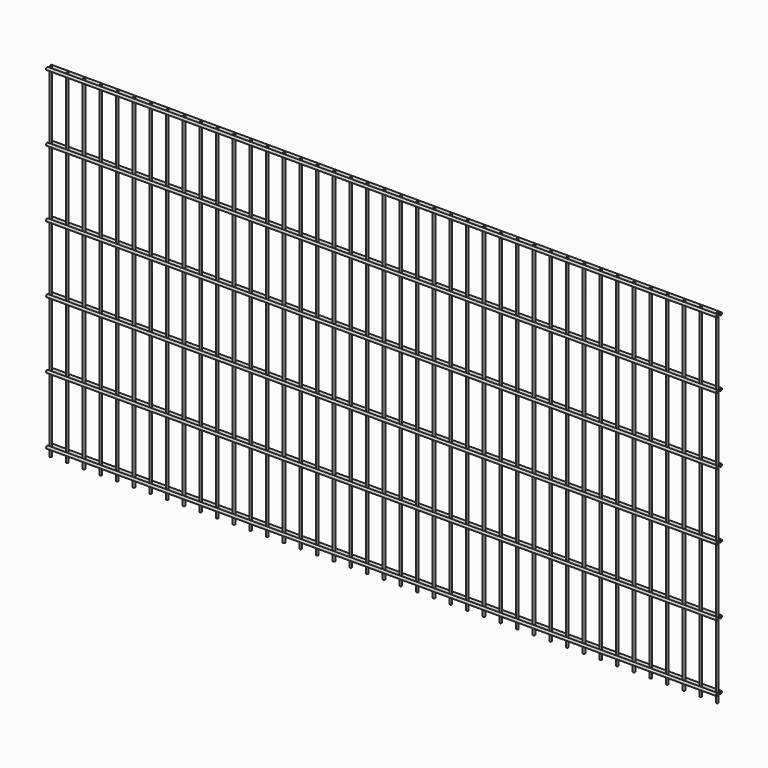
from build123d import *

# Parameters (mm, degrees)
F0_R     = 3
F1_DEPTH = 1030
F2_R     = 4
F3_DEPTH = 1005


with BuildPart() as f1:
    # F0 (on Top) → F1 (new body)
    with BuildSketch(Plane.XY):
        with Locations((750, 0)):
            Circle(F0_R)
    extrude(amount=-F1_DEPTH)


with BuildPart() as f1b:
    # F0 (on Top) → F1, piece 2 (new body)
    with BuildSketch(Plane.XY):
        with Locations((-550, 0)):
            Circle(F0_R)
    extrude(amount=-F1_DEPTH)


with BuildPart() as f1c:
    # F0 (on Top) → F1, piece 3 (new body)
    with BuildSketch(Plane.XY):
        with Locations((950, 0)):
            Circle(F0_R)
    extrude(amount=-F1_DEPTH)


with BuildPart() as f1d:
    # F0 (on Top) → F1, piece 4 (new body)
    with BuildSketch(Plane.XY):
        with Locations((450, 0)):
            Circle(F0_R)
    extrude(amount=-F1_DEPTH)


with BuildPart() as f1e:
    # F0 (on Top) → F1, piece 5 (new body)
    with BuildSketch(Plane.XY):
        with Locations((-800, 0)):
            Circle(F0_R)
    extrude(amount=-F1_DEPTH)


with BuildPart() as f1f:
    # F0 (on Top) → F1, piece 6 (new body)
    with BuildSketch(Plane.XY):
        with Locations((-900, 0)):
            Circle(F0_R)
    extrude(amount=-F1_DEPTH)


with BuildPart() as f1g:
    # F0 (on Top) → F1, piece 7 (new body)
    with BuildSketch(Plane.XY):
        with Locations((350, 0)):
            Circle(F0_R)
    extrude(amount=-F1_DEPTH)


with BuildPart() as f1h:
    # F0 (on Top) → F1, piece 8 (new body)
    with BuildSketch(Plane.XY):
        with Locations((-700, 0)):
            Circle(F0_R)
    extrude(amount=-F1_DEPTH)


with BuildPart() as f1i:
    # F0 (on Top) → F1, piece 9 (new body)
    with BuildSketch(Plane.XY):
        with Locations((1000, 0)):
            Circle(F0_R)
    extrude(amount=-F1_DEPTH)


with BuildPart() as f1j:
    # F0 (on Top) → F1, piece 10 (new body)
    with BuildSketch(Plane.XY):
        with Locations((600, 0)):
            Circle(F0_R)
    extrude(amount=-F1_DEPTH)


with BuildPart() as f1k:
    # F0 (on Top) → F1, piece 11 (new body)
    with BuildSketch(Plane.XY):
        with Locations((700, 0)):
            Circle(F0_R)
    extrude(amount=-F1_DEPTH)


with BuildPart() as f1l:
    # F0 (on Top) → F1, piece 12 (new body)
    with BuildSketch(Plane.XY):
        with Locations((650, 0)):
            Circle(F0_R)
    extrude(amount=-F1_DEPTH)


with BuildPart() as f1m:
    # F0 (on Top) → F1, piece 13 (new body)
    with BuildSketch(Plane.XY):
        with Locations((-650, 0)):
            Circle(F0_R)
    extrude(amount=-F1_DEPTH)


with BuildPart() as f1n:
    # F0 (on Top) → F1, piece 14 (new body)
    with BuildSketch(Plane.XY):
        with Locations((850, 0)):
            Circle(F0_R)
    extrude(amount=-F1_DEPTH)


with BuildPart() as f1o:
    # F0 (on Top) → F1, piece 15 (new body)
    with BuildSketch(Plane.XY):
        with Locations((-300, 0)):
            Circle(F0_R)
    extrude(amount=-F1_DEPTH)


with BuildPart() as f1p:
    # F0 (on Top) → F1, piece 16 (new body)
    with BuildSketch(Plane.XY):
        with Locations((-250, 0)):
            Circle(F0_R)
    extrude(amount=-F1_DEPTH)


with BuildPart() as f1q:
    # F0 (on Top) → F1, piece 17 (new body)
    with BuildSketch(Plane.XY):
        with Locations((-350, 0)):
            Circle(F0_R)
    extrude(amount=-F1_DEPTH)


with BuildPart() as f1r:
    # F0 (on Top) → F1, piece 18 (new body)
    with BuildSketch(Plane.XY):
        with Locations((-400, 0)):
            Circle(F0_R)
    extrude(amount=-F1_DEPTH)


with BuildPart() as f1s:
    # F0 (on Top) → F1, piece 19 (new body)
    with BuildSketch(Plane.XY):
        with Locations((-500, 0)):
            Circle(F0_R)
    extrude(amount=-F1_DEPTH)


with BuildPart() as f1t:
    # F0 (on Top) → F1, piece 20 (new body)
    with BuildSketch(Plane.XY):
        with Locations((-950, 0)):
            Circle(F0_R)
    extrude(amount=-F1_DEPTH)


with BuildPart() as f1u:
    # F0 (on Top) → F1, piece 21 (new body)
    with BuildSketch(Plane.XY):
        with Locations((-450, 0)):
            Circle(F0_R)
    extrude(amount=-F1_DEPTH)


with BuildPart() as f1v:
    # F0 (on Top) → F1, piece 22 (new body)
    with BuildSketch(Plane.XY):
        with Locations((150, 0)):
            Circle(F0_R)
    extrude(amount=-F1_DEPTH)


with BuildPart() as f1w:
    # F0 (on Top) → F1, piece 23 (new body)
    with BuildSketch(Plane.XY):
        with Locations((50, 0)):
            Circle(F0_R)
    extrude(amount=-F1_DEPTH)


with BuildPart() as f1x:
    # F0 (on Top) → F1, piece 24 (new body)
    with BuildSketch(Plane.XY):
        with Locations((100, 0)):
            Circle(F0_R)
    extrude(amount=-F1_DEPTH)


with BuildPart() as f1y:
    # F0 (on Top) → F1, piece 25 (new body)
    with BuildSketch(Plane.XY):
        Circle(F0_R)
    extrude(amount=-F1_DEPTH)


with BuildPart() as f1z:
    # F0 (on Top) → F1, piece 26 (new body)
    with BuildSketch(Plane.XY):
        with Locations((-50, 0)):
            Circle(F0_R)
    extrude(amount=-F1_DEPTH)


with BuildPart() as f1ba:
    # F0 (on Top) → F1, piece 27 (new body)
    with BuildSketch(Plane.XY):
        with Locations((-150, 0)):
            Circle(F0_R)
    extrude(amount=-F1_DEPTH)


with BuildPart() as f1bb:
    # F0 (on Top) → F1, piece 28 (new body)
    with BuildSketch(Plane.XY):
        with Locations((-100, 0)):
            Circle(F0_R)
    extrude(amount=-F1_DEPTH)


with BuildPart() as f1bc:
    # F0 (on Top) → F1, piece 29 (new body)
    with BuildSketch(Plane.XY):
        with Locations((-1000, 0)):
            Circle(F0_R)
    extrude(amount=-F1_DEPTH)


with BuildPart() as f1bd:
    # F0 (on Top) → F1, piece 30 (new body)
    with BuildSketch(Plane.XY):
        with Locations((300, 0)):
            Circle(F0_R)
    extrude(amount=-F1_DEPTH)


with BuildPart() as f1be:
    # F0 (on Top) → F1, piece 31 (new body)
    with BuildSketch(Plane.XY):
        with Locations((250, 0)):
            Circle(F0_R)
    extrude(amount=-F1_DEPTH)


with BuildPart() as f1bf:
    # F0 (on Top) → F1, piece 32 (new body)
    with BuildSketch(Plane.XY):
        with Locations((-200, 0)):
            Circle(F0_R)
    extrude(amount=-F1_DEPTH)


with BuildPart() as f1bg:
    # F0 (on Top) → F1, piece 33 (new body)
    with BuildSketch(Plane.XY):
        with Locations((900, 0)):
            Circle(F0_R)
    extrude(amount=-F1_DEPTH)


with BuildPart() as f1bh:
    # F0 (on Top) → F1, piece 34 (new body)
    with BuildSketch(Plane.XY):
        with Locations((-750, 0)):
            Circle(F0_R)
    extrude(amount=-F1_DEPTH)


with BuildPart() as f1bi:
    # F0 (on Top) → F1, piece 35 (new body)
    with BuildSketch(Plane.XY):
        with Locations((200, 0)):
            Circle(F0_R)
    extrude(amount=-F1_DEPTH)


with BuildPart() as f1bj:
    # F0 (on Top) → F1, piece 36 (new body)
    with BuildSketch(Plane.XY):
        with Locations((500, 0)):
            Circle(F0_R)
    extrude(amount=-F1_DEPTH)


with BuildPart() as f1bk:
    # F0 (on Top) → F1, piece 37 (new body)
    with BuildSketch(Plane.XY):
        with Locations((550, 0)):
            Circle(F0_R)
    extrude(amount=-F1_DEPTH)


with BuildPart() as f1bl:
    # F0 (on Top) → F1, piece 38 (new body)
    with BuildSketch(Plane.XY):
        with Locations((-600, 0)):
            Circle(F0_R)
    extrude(amount=-F1_DEPTH)


with BuildPart() as f1bm:
    # F0 (on Top) → F1, piece 39 (new body)
    with BuildSketch(Plane.XY):
        with Locations((800, 0)):
            Circle(F0_R)
    extrude(amount=-F1_DEPTH)


with BuildPart() as f1bn:
    # F0 (on Top) → F1, piece 40 (new body)
    with BuildSketch(Plane.XY):
        with Locations((-850, 0)):
            Circle(F0_R)
    extrude(amount=-F1_DEPTH)


with BuildPart() as f1bo:
    # F0 (on Top) → F1, piece 41 (new body)
    with BuildSketch(Plane.XY):
        with Locations((400, 0)):
            Circle(F0_R)
    extrude(amount=-F1_DEPTH)


with BuildPart() as f3:
    # F2 (on Right) → F3 (new body, symmetric)
    with BuildSketch(Plane.YZ):
        with Locations((7, -4)):
            Circle(F2_R)
    extrude(amount=F3_DEPTH, both=True)


with BuildPart() as f3b:
    # F2 (on Right) → F3, piece 2 (new body, symmetric)
    with BuildSketch(Plane.YZ):
        with Locations((-7, -4)):
            Circle(F2_R)
    extrude(amount=F3_DEPTH, both=True)


with BuildPart() as f3c:
    # F2 (on Right) → F3, piece 3 (new body, symmetric)
    with BuildSketch(Plane.YZ):
        with Locations((7, -204)):
            Circle(F2_R)
    extrude(amount=F3_DEPTH, both=True)


with BuildPart() as f3d:
    # F2 (on Right) → F3, piece 4 (new body, symmetric)
    with BuildSketch(Plane.YZ):
        with Locations((-7, -204)):
            Circle(F2_R)
    extrude(amount=F3_DEPTH, both=True)


with BuildPart() as f3e:
    # F2 (on Right) → F3, piece 5 (new body, symmetric)
    with BuildSketch(Plane.YZ):
        with Locations((7, -404)):
            Circle(F2_R)
    extrude(amount=F3_DEPTH, both=True)


with BuildPart() as f3f:
    # F2 (on Right) → F3, piece 6 (new body, symmetric)
    with BuildSketch(Plane.YZ):
        with Locations((-7, -404)):
            Circle(F2_R)
    extrude(amount=F3_DEPTH, both=True)


with BuildPart() as f3g:
    # F2 (on Right) → F3, piece 7 (new body, symmetric)
    with BuildSketch(Plane.YZ):
        with Locations((7, -604)):
            Circle(F2_R)
    extrude(amount=F3_DEPTH, both=True)


with BuildPart() as f3h:
    # F2 (on Right) → F3, piece 8 (new body, symmetric)
    with BuildSketch(Plane.YZ):
        with Locations((-7, -604)):
            Circle(F2_R)
    extrude(amount=F3_DEPTH, both=True)


with BuildPart() as f3i:
    # F2 (on Right) → F3, piece 9 (new body, symmetric)
    with BuildSketch(Plane.YZ):
        with Locations((7, -804)):
            Circle(F2_R)
    extrude(amount=F3_DEPTH, both=True)


with BuildPart() as f3j:
    # F2 (on Right) → F3, piece 10 (new body, symmetric)
    with BuildSketch(Plane.YZ):
        with Locations((-7, -804)):
            Circle(F2_R)
    extrude(amount=F3_DEPTH, both=True)


with BuildPart() as f3k:
    # F2 (on Right) → F3, piece 11 (new body, symmetric)
    with BuildSketch(Plane.YZ):
        with Locations((7, -1004)):
            Circle(F2_R)
    extrude(amount=F3_DEPTH, both=True)


with BuildPart() as f3l:
    # F2 (on Right) → F3, piece 12 (new body, symmetric)
    with BuildSketch(Plane.YZ):
        with Locations((-7, -1004)):
            Circle(F2_R)
    extrude(amount=F3_DEPTH, both=True)


solid = Compound([f1.part, f1b.part, f1c.part, f1d.part, f1e.part, f1f.part, f1g.part, f1h.part, f1i.part, f1j.part, f1k.part, f1l.part, f1m.part, f1n.part, f1o.part, f1p.part, f1q.part, f1r.part, f1s.part, f1t.part, f1u.part, f1v.part, f1w.part, f1x.part, f1y.part, f1z.part, f1ba.part, f1bb.part, f1bc.part, f1bd.part, f1be.part, f1bf.part, f1bg.part, f1bh.part, f1bi.part, f1bj.part, f1bk.part, f1bl.part, f1bm.part, f1bn.part, f1bo.part, f3.part, f3b.part, f3c.part, f3d.part, f3e.part, f3f.part, f3g.part, f3h.part, f3i.part, f3j.part, f3k.part, f3l.part])
